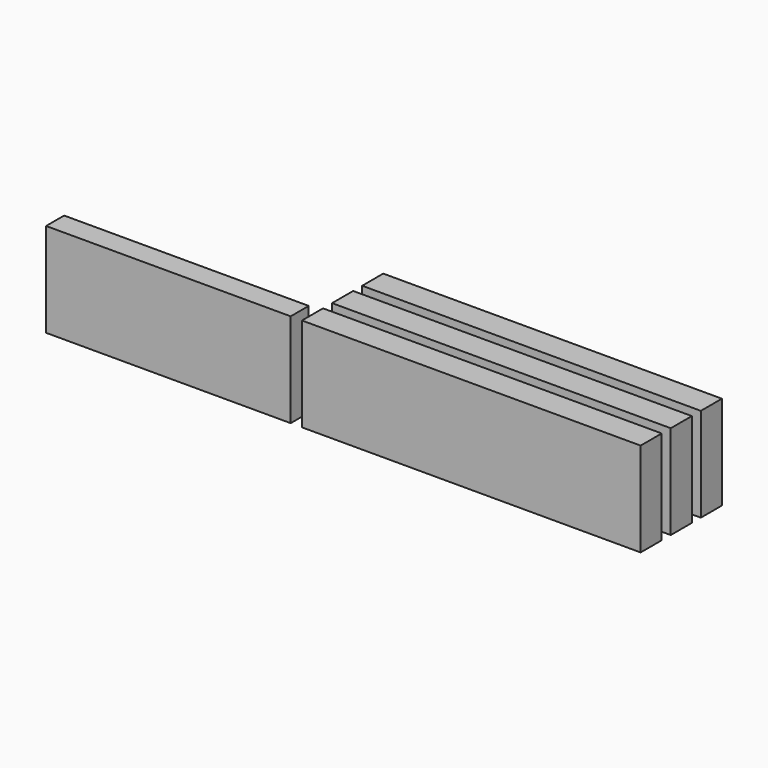
from build123d import *

# Parameters (mm, degrees)
F0_W     = 90
F0_H     = 7
F1_DEPTH = 25
F0_W_2   = 65
F0_H_2   = 6
F2_DEPTH = 25


# Not quite as in the source:
# - a feature names something its author has since deleted; it is built from what else it names


with BuildPart() as f1:
    # F0 (on Top) → F1 (new body)
    with BuildSketch(Plane.XY):
        with Locations((-4.7864606604, 1.3194340005)):
            Rectangle(F0_W, F0_H)
    extrude(amount=F1_DEPTH)


with BuildPart() as f1b:
    # F0 (on Top) → F1, piece 2 (new body)
    with BuildSketch(Plane.XY):
        Polygon((40.2135393396, -5.1805659995), (-49.7864606604, -5.1805659995), (-49.7864606604, -12.1805659995), (15.2135393396, -12.1805659995), (40.2135393396, -12.1805659995), align=None)
    extrude(amount=F1_DEPTH)

    # F0 (on Top) → F2, piece 2 (join)
    with BuildSketch(Plane.XY):
        Polygon((40.2135393396, -5.1805659995), (-49.7864606604, -5.1805659995), (-49.7864606604, -12.1805659995), (15.2135393396, -12.1805659995), (40.2135393396, -12.1805659995), align=None)
    extrude(amount=F2_DEPTH)


with BuildPart() as f1c:
    # F0 (on Top) → F1, piece 3 (new body)
    with BuildSketch(Plane.XY):
        with Locations((-85.2864606604, -9.1805659995)):
            Rectangle(F0_W_2, F0_H_2)
    extrude(amount=F1_DEPTH)


with BuildPart() as f2:
    # F0 (on Top) → F2 (new body)
    with BuildSketch(Plane.XY):
        with Locations((-4.7864606604, 11.3194340005)):
            Rectangle(F0_W, F0_H)
    extrude(amount=F2_DEPTH)


solid = Compound([f1.part, f1b.part, f1c.part, f2.part])
